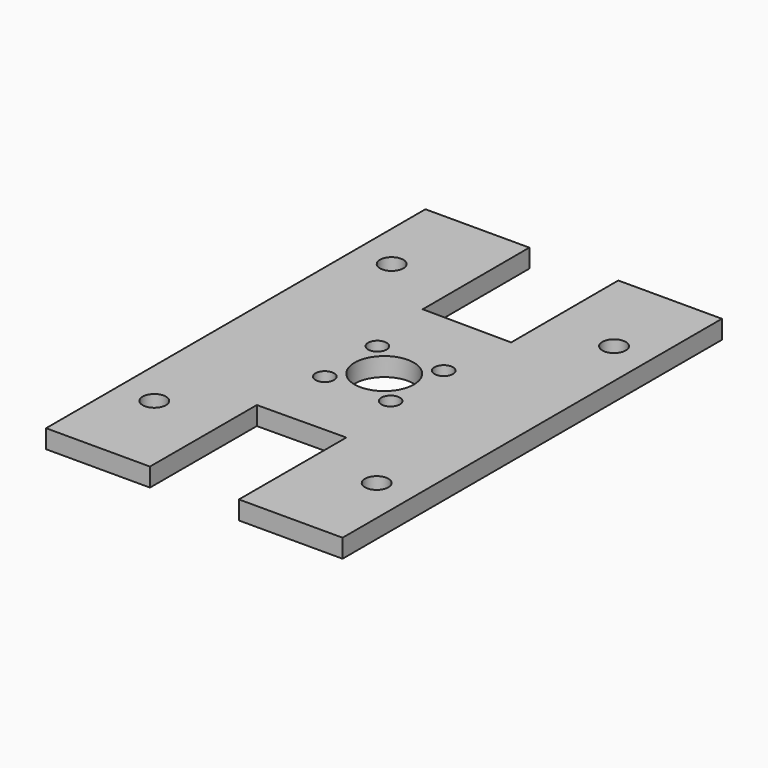
from build123d import *

# Parameters (mm, degrees)
F0_R     = 2
F0_R_2   = 1.5875
F0_R_3   = 5.08
F1_DEPTH = 3.175


# Not quite as in the source:
# - a feature names something its author has since deleted; it is built from what else it names


with BuildPart() as f1:
    # F0 (on Top) → F1 (new body)
    with BuildSketch(Plane.XY):
        Polygon((-25.4426629463, 106.7507229011), (-25.4426629463, 25.5024298209), (-7.6439069871, 25.5024298209), (-7.6197668711, 48.3624170749), (7.6197668654, 48.4816290427), (7.5955008617, 25.5024298209), (25.3573370537, 25.5024298209), (25.3573370537, 106.7507229011), (7.5955008617, 106.7507229011), (7.6197668654, 83.7715236793), (-7.6197668711, 83.8907356471), (-7.6439069871, 106.7507229011), align=None)
        with Locations((-19.0798602959, 40.726575638)):
            Circle(F0_R, mode=Mode.SUBTRACT)
        with Locations((-5.6575617589, 60.4690146843)):
            Circle(F0_R_2, mode=Mode.SUBTRACT)
        with Locations((19.0201352736, 40.726576361)):
            Circle(F0_R, mode=Mode.SUBTRACT)
        with Locations((5.6336971198, 60.4452502854)):
            Circle(F0_R_2, mode=Mode.SUBTRACT)
        with Locations((0, 66.126575638)):
            Circle(F0_R_3, mode=Mode.SUBTRACT)
        with Locations((-5.6815269438, 71.7600694551)):
            Circle(F0_R_2, mode=Mode.SUBTRACT)
        with Locations((-19.05, 91.526576114)):
            Circle(F0_R, mode=Mode.SUBTRACT)
        with Locations((5.6815266776, 71.7600697236)):
            Circle(F0_R_2, mode=Mode.SUBTRACT)
        with Locations((19.05, 91.526576361)):
            Circle(F0_R, mode=Mode.SUBTRACT)
    extrude(amount=F1_DEPTH)


solid = f1.part
